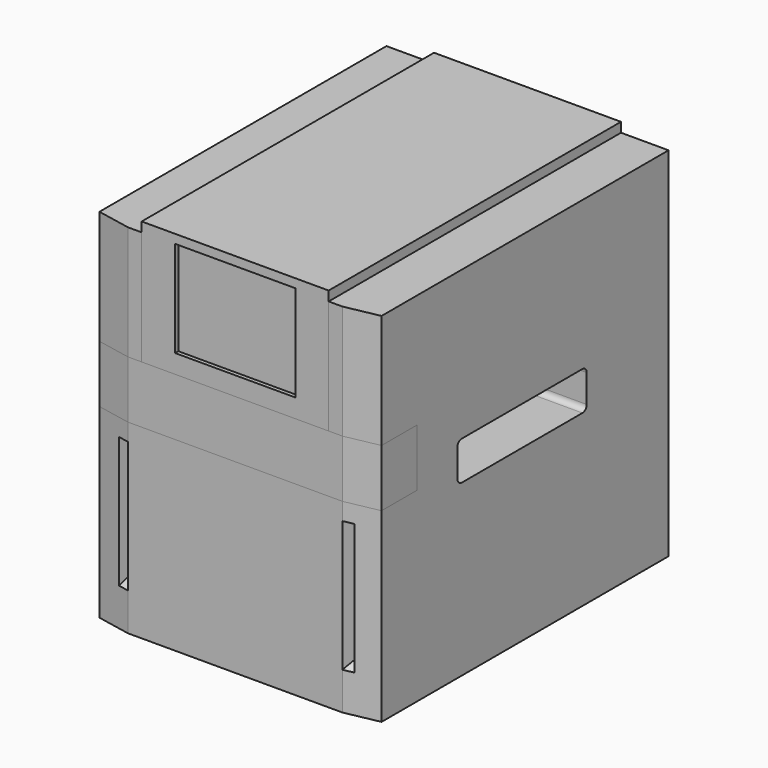
from build123d import *

# Parameters (mm, degrees)
F1_DEPTH     = 1338
F3_DEPTH     = 642
F4_DEPTH     = 215
F5_W         = 700
F5_H         = 190
F6_DEPTH     = 463
F8_DEPTH     = 427
F9_W         = 700
F9_H         = 36
F10_DEPTH    = 1178
F11_W        = 605
F11_H        = 145
F12_DEPTH    = 1056.001
F13_R        = 20
F14_W        = 450
F14_H        = 360
F15_DEPTH    = 25
F16_DEPTH    = 10
F17_W        = 40
F17_H        = 490
F18_DEPTH    = 40
F19_SIZE2    = 19.99999
F19_SIZE     = 39.99999
F20_W        = 40
F20_H        = 490
F21_DEPTH    = 40
F22_T1_DEPTH = 593.5931549515
F22_T3_DEPTH = 40
F22_T5_DEPTH = 40


# Not quite as in the source:
# - a fillet or chamfer that OpenCascade refuses, or shapes differently, is made with other operations: its cross-section is extruded or revolved along the edge and cut away or added
# - a fillet or chamfer is up to 0.001 mm smaller than in the source, because OpenCascade refuses the exact size


with BuildPart() as f1:
    # F0 (on Top) → F1 (new body)
    with BuildSketch(Plane.XY):
        Polygon((1056, 1368), (0, 1368), (0, 25), (126.5, 0), (929.5, 0), (1056, 25), align=None)
    extrude(amount=F1_DEPTH)

    # F2 (on face) → F3 (cut)
    with BuildSketch(Plane.XY.offset(1338)):
        Polygon((1056, 190), (0, 190), (0, 25), (126.5, 0), (929.5, 0), (1056, 25), align=None)
    extrude(amount=-F3_DEPTH, mode=Mode.SUBTRACT)


with BuildPart() as f4:
    # F4 (new): a face of the model
    f4_faces = [f1.part.faces().sort_by_distance(p)[0] for p in [
        (528, 96.3879218308, 696),
    ]]
    extrude(f4_faces, amount=F4_DEPTH)


with BuildPart() as f6:
    # F5 (on face) → F6 (new body)
    with BuildSketch(Plane.XY.offset(911)):
        with Locations((528, 95)):
            Rectangle(F5_W, F5_H)
    extrude(amount=F6_DEPTH)

    # F9 (on face) → F10 (join, through all)
    with BuildSketch(Plane(origin=(0, 190, 0), x_dir=(-1, 0, 0), z_dir=(0, 1, 0))):
        with Locations((-528, 1356)):
            Rectangle(F9_W, F9_H)
    extrude(amount=F10_DEPTH)

    # F14 (on face) → F15 (cut)
    with BuildSketch(Plane.XZ):
        with Locations((528, 1161)):
            Rectangle(F14_W, F14_H)
    extrude(amount=-F15_DEPTH, mode=Mode.SUBTRACT)


with BuildPart() as f1_1:
    add(f1.part)

    # F7 (on face) → F8 (join, through all)
    with BuildSketch(Plane.XY.offset(911)):
        Polygon((0, 25), (126.5, 0), (178, 0), (178, 190), (0, 190), align=None)
        Polygon((878, 190), (878, 0), (929.5, 0), (1056, 25), (1056, 190), align=None)
    extrude(amount=F8_DEPTH)

    # F11 (on face) → F12 (cut, through all)
    with BuildSketch(Plane.YZ.offset(1056)):
        with Locations((682.5, 708.5)):
            Rectangle(F11_W, F11_H)
    extrude(amount=-F12_DEPTH, mode=Mode.SUBTRACT)

    # F13
    f13_edges = [f1_1.edges().sort_by_distance(p)[0] for p in [
        (528, 380, 781),
        (528, 985, 781),
        (528, 380, 636),
        (528, 985, 636),
    ]]
    fillet(f13_edges, radius=F13_R)

    # F17 (on face) → F18 (cut)
    with BuildSketch(Plane(origin=(4.7549955645, 24.0602775564, 0), x_dir=(0.981025536, -0.1938785644, 0), z_dir=(-0.1938785644, -0.981025536, 0))):
        with Locations((104.0997303022, 386)):
            Rectangle(F17_W, F17_H)
    extrude(amount=-F18_DEPTH, mode=Mode.SUBTRACT)

    # F19 (size 40 and 20 in the source; OpenCascade refuses exactly that, so slightly less here)
    f19_edges = [f1_1.edges().sort_by_distance(p)[0] for p in [
        (134.255143, 39.241021, 386),
        (114.634632, 43.118593, 631),
        (114.634632, 43.118593, 141),
    ]]
    chamfer(f19_edges, length=F19_SIZE, length2=F19_SIZE2)

    # F20 (on face) → F21 (cut)
    with BuildSketch(Plane(origin=(34.9388804523, -176.7907350885, 0), x_dir=(0.981025536, 0.1938785644, 0), z_dir=(0.1938785644, -0.981025536, 0))):
        with Locations((931.8632356991, 386)):
            Rectangle(F20_W, F20_H)
    extrude(amount=-F21_DEPTH, mode=Mode.SUBTRACT)

    # F22: chamfer of 20 x 40 on 3 edges, made by hand

    # F22_s2 → F22_t1 (join)
    with BuildSketch(Plane.XY.offset(37.4068450485)):
        Polygon((929.5, 0), (941.3653681428, 43.1185927279), (921.744857423, 39.2410214394), align=None)
    extrude(amount=F22_T1_DEPTH)

    # F22_s4 → F22_t3 (join)
    with BuildSketch(Plane(origin=(933.8021409872, 184.5458776655, 0), x_dir=(0, 0, 1), z_dir=(-0.981025536, -0.1938785644, 0))):
        Polygon((631, -180.2101256322), (611, -140.2101256322), (631, -140.2101256322), align=None)
    extrude(amount=F22_T3_DEPTH)

    # F22_s6 → F22_t5 (join)
    with BuildSketch(Plane(origin=(894.5611195477, 176.7907350885, 0), x_dir=(0, 0, 1), z_dir=(0.981025536, 0.1938785644, 0))):
        Polygon((141, 180.2101256322), (161, 140.2101256322), (141, 140.2101256322), align=None)
    extrude(amount=F22_T5_DEPTH)


with BuildPart() as f16:
    # F16 (new): a face of the model
    f16_faces = [f6.part.faces().sort_by_distance(p)[0] for p in [
        (528, 25, 1161),
    ]]
    extrude(f16_faces, amount=F16_DEPTH)


solid = Compound([f4.part, f6.part, f1_1.part, f16.part])
